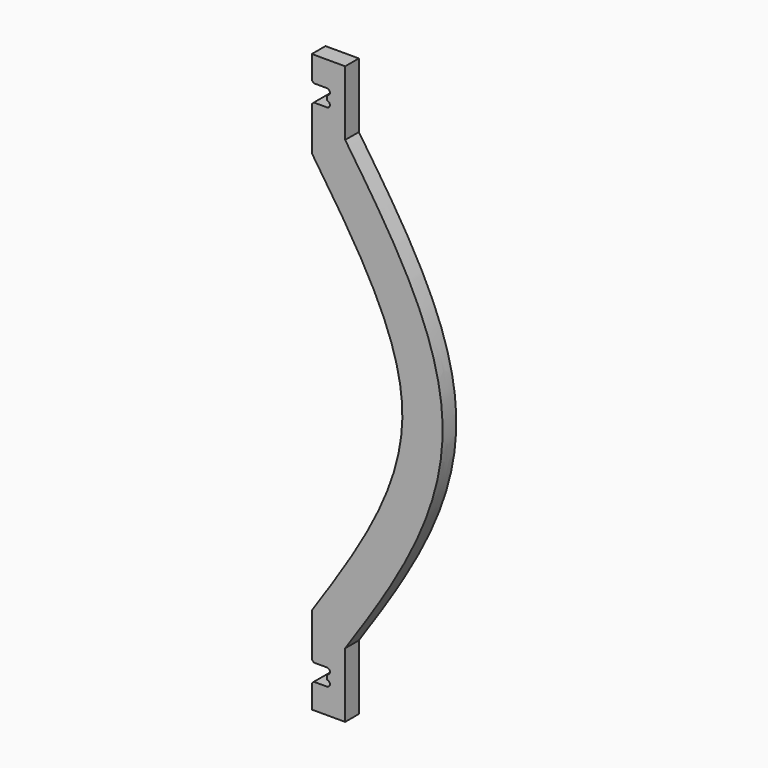
from build123d import *

# Parameters (mm, degrees)
F1_DEPTH = 17
F2_R     = 3
F3_DEPTH = 25
F4_SIZE  = 2


# Not quite as in the source:
# - the dataset's text gives a spline's control points without its knots; the knots are read off the source's solid


with BuildPart() as f1:
    # F0 (on Front) → F1 (new body)
    with BuildSketch(Plane.XZ):
        with BuildLine():
            Line((0, 245), (0, 200))
            add(Edge.make_bspline(
                [(0, 200), (45, 133.3333333333), (135, 0), (45, -133.3333333333), (0, -200)],
                knots=[0, 0, 0, 0, 0.5, 1, 1, 1, 1], degree=3))
            Line((0, -200), (0, -245))
            Line((0, -245), (15, -245))
            Line((15, -245), (15, -261.8))
            Line((15, -261.8), (0, -261.8))
            Line((0, -261.8), (0, -286.8))
            Line((0, -286.8), (33.153946963, -286.8))
            Line((33.153946963, -286.8), (33.153946963, -222.3789142))
            add(Edge.make_bspline(
                [(33.153946963, 222.3789142), (38.778946963, 214.0455808667), (50.1370946994, 197.2199375913), (66.9704607705, 171.4834064893), (83.0666221963, 145.1835388594), (97.8752152805, 118.2069155881), (108.6517536257, 95.0256105135), (115.9962383389, 75.9610643166), (120.768213582, 61.3791709128), (124.6977896579, 46.4952551717), (127.1729613057, 33.8331492243), (128.6105780855, 23.5524512191), (129.4012955844, 15.7700211508), (129.8071764378, 9.2278748435), (129.9720929215, 3.9649278514), (130.0139535392, 0), (129.9720929215, -3.9649278514), (129.8071764378, -9.2278748435), (129.4012955844, -15.7700211508), (128.6105780855, -23.5524512191), (127.1729613057, -33.8331492243), (124.6977896579, -46.4952551717), (120.768213582, -61.3791709128), (115.9962383389, -75.9610643166), (108.6517536257, -95.0256105135), (97.8752152805, -118.2069155881), (83.0666221963, -145.1835388594), (66.9704607705, -171.4834064893), (50.1370946994, -197.2199375913), (38.778946963, -214.0455808667), (33.153946963, -222.3789142)],
                knots=[0, 0, 0, 0, 0.0625, 0.125, 0.1875, 0.25, 0.3125, 0.34375, 0.375, 0.40625, 0.4375, 0.453125, 0.46875, 0.484375, 0.4921875, 0.5, 0.5078125, 0.515625, 0.53125, 0.546875, 0.5625, 0.59375, 0.625, 0.65625, 0.6875, 0.75, 0.8125, 0.875, 0.9375, 1, 1, 1, 1], degree=3))
            Line((33.153946963, 222.3789142), (33.153946963, 286.8))
            Line((33.153946963, 286.8), (0, 286.8))
            Line((0, 286.8), (0, 261.8))
            Line((0, 261.8), (15, 261.8))
            Line((15, 261.8), (15, 245))
            Line((15, 245), (0, 245))
        make_face()
    extrude(amount=F1_DEPTH)

    # F2 (on face) → F3 (cut)
    with BuildSketch(Plane.XZ.offset(17)):
        with Locations((15, 248)):
            Circle(F2_R)
        with Locations((15, 258.8)):
            Circle(F2_R)
        with Locations((15, -248)):
            Circle(F2_R)
        with Locations((15, -258.8)):
            Circle(F2_R)
    extrude(amount=-F3_DEPTH, mode=Mode.SUBTRACT)

    # F4
    f4_edges = [f1.edges().sort_by_distance(p)[0] for p in [
        (0, -8.5, 261.8),
        (0, -8.5, 245),
        (0, -8.5, -245),
        (0, -8.5, -261.8),
    ]]
    chamfer(f4_edges, length=F4_SIZE)


solid = f1.part
